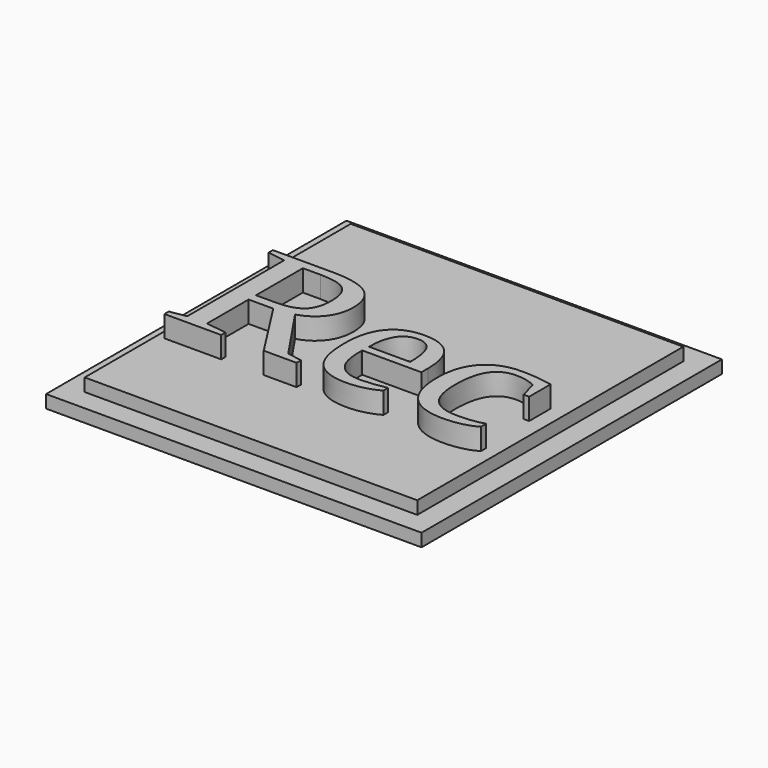
from build123d import *

# Parameters (mm, degrees)
F0_W         = 35
F0_H         = 35
F1_DEPTH     = 1.2
F2_W         = 31
F2_H         = 31
F3_DEPTH     = 1.2
F4_TEXT_SIZE = 19.5390978925
F5_DEPTH     = 2


# Not quite as in the source:
# - Text() gives the source's letters only with a copy of the font that has no kerning and outlines rounded to 1/6400 em; it was checked with that copy


with BuildPart() as f1:
    # F0 (on Top) → F1 (new body)
    with BuildSketch(Plane.XY):
        with Locations((17.5, 17.5)):
            Rectangle(F0_W, F0_H)
    extrude(amount=F1_DEPTH)

    # F2 (on face) → F3 (join)
    with BuildSketch(Plane.XY.offset(1.2)):
        with Locations((17.5, 17.5)):
            Rectangle(F2_W, F2_H)
    extrude(amount=F3_DEPTH)

    # F4 (on face) → F5 (join)
    with BuildSketch(Plane.XY.offset(2.4)):
        with Locations((2, 10.4318495174)):
            Text('Rec', F4_TEXT_SIZE, font='Tinos', text_align=(TextAlign.LEFT, TextAlign.BOTTOM))
    extrude(amount=F5_DEPTH)


solid = f1.part
